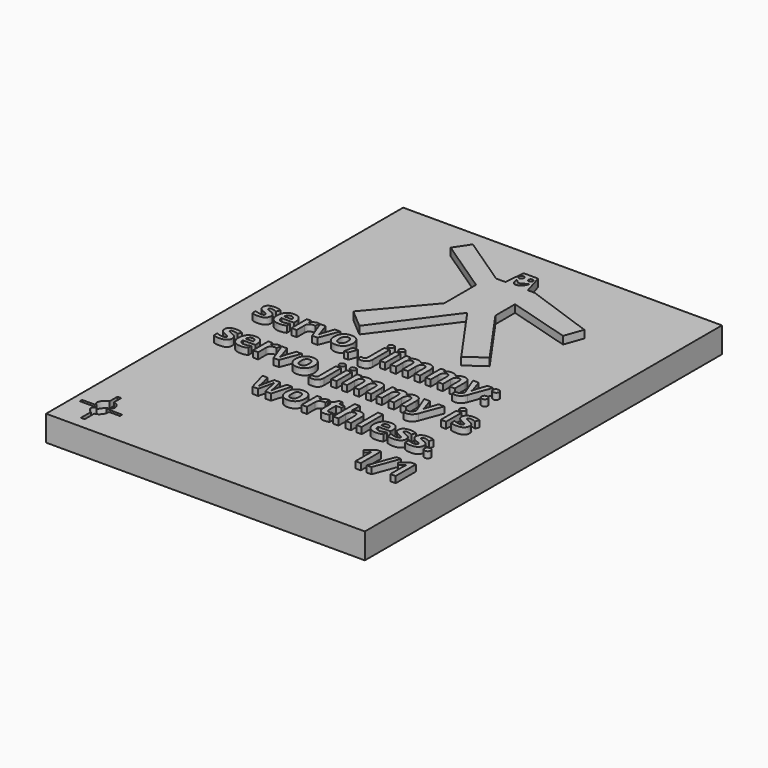
from build123d import *

# Parameters (mm, degrees)
F0_W         = 63.5
F0_H         = 88.9
F1_DEPTH     = 5.08
F2_R         = 0.483936804
F2_R_2       = 0.4231425129
F3_DEPTH     = 1.524
F5_DEPTH     = 1.27
F6_TEXT_SIZE = 7.0555555556
F7_DEPTH     = 1.27


# Not quite as in the source:
# - Text() gives the source's letters only with a copy of the font that has no kerning and outlines rounded to 1/6400 em; it was checked with that copy


with BuildPart() as f1:
    # F0 (on Top) → F1 (new body)
    with BuildSketch(Plane.XY):
        Rectangle(F0_W, F0_H)
    extrude(amount=F1_DEPTH)

    # F2 (on face) → F3 (join)
    with BuildSketch(Plane.XY.offset(5.08)):
        Polygon((-10.3656723576, 6.8217876206), (0, 20.7275711), (8.5247382522, 8.577182889), (12.1481206254, 11.1193556807), (4.0015474354, 22.7307417338), (4.0015474354, 27.6327357116), (4.0015474354, 32.5347296894), (2.6223212481, 32.5347296894), (0, 32.5347296894), (-1.8471479416, 32.5347296894), (-3.6942958832, 32.5347296894), (-13.7166529894, 39.2620638013), (-15.7326752015, 36.2586014777), (-4.7968987376, 28.9181503975), (-4.7968987376, 21.0021585226), (-14.1285285354, 10.0187547505), align=None)
        Polygon((4.0015474354, 32.5347296894), (4.0015474354, 27.6327357116), (16.4861305487, 23.9590620018), (17.7919864655, 27.6327357116), align=None)
        Polygon((0, 32.5347296894), (2.6223212481, 32.5347296894), (1.399056986, 36.6094112396), (0, 36.6094112396), (-1.4804843813, 36.6094112396), (-1.8471479416, 32.5347296894), align=None)
        with Locations((-0.8866756689, 35.3195294738)):
            Circle(F2_R, mode=Mode.SUBTRACT)
        with BuildLine():
            add(Edge.make_bspline(
                [(-0.8501152042, 34.1562442482), (-0.7343137138, 34.1961865805), (-0.0467516661, 32.880225173), (1.9143940204, 35.0437316808), (1.0316503155, 32.8797391223), (-0.7778123329, 32.509153736), (-0.9740249003, 34.1135052277), (-0.8501152042, 34.1562442482)],
                knots=[0, 0, 0, 0, 0.1780613573, 0.4016291559, 0.5959136983, 0.8094711166, 1, 1, 1, 1], degree=3))
        make_face(mode=Mode.SUBTRACT)
        with Locations((0.9081121534, 35.3893265128)):
            Circle(F2_R_2, mode=Mode.SUBTRACT)
    extrude(amount=F3_DEPTH)

    # F4 (on face) → F5 (cut)
    with BuildSketch(Plane.XY.offset(5.08)):
        with BuildLine():
            add(Edge.make_bspline(
                [(-25.6292883469, -37.4438245498), (-25.5440439647, -37.4063721569), (-25.4620471143, -37.3631067403), (-25.3843005295, -37.3148079962)],
                knots=[0.0680076943, 0.0680076943, 0.0680076943, 0.0680076943, 0.0966302435, 0.0966302435, 0.0966302435, 0.0966302435], degree=3))
            add(Edge.make_bspline(
                [(-25.6292883469, -37.4438245498), (-25.2227961776, -37.3837119487), (-24.7132209679, -37.4270308297), (-24.5209995881, -37.774670522), (-24.4905924923, -37.8889460117)],
                knots=[0.0689407267, 0.0689407267, 0.0689407267, 0.0689407267, 0.2018413649, 0.2544963619, 0.2544963619, 0.2544963619, 0.2544963619], degree=3))
            Line((-24.4905924923, -37.8889460117), (-22.2920402884, -37.8889460117))
            Line((-22.2920402884, -37.8889460117), (-22.2920402884, -37.3148079962))
            Line((-22.2920402884, -37.3148079962), (-25.3843005295, -37.3148079962))
        make_face()
        with BuildLine():
            Line((-26.6530141234, -37.5985746456), (-26.6530141234, -37.5851999525))
            add(Edge.make_bspline(
                [(-27.4060703076, -37.3148079962), (-27.1886195833, -37.4508936414), (-26.9254983415, -37.5462389939), (-26.6530141234, -37.5851999525)],
                knots=[0.8801095423, 0.8801095423, 0.8801095423, 0.8801095423, 0.9624938443, 0.9624938443, 0.9624938443, 0.9624938443], degree=3))
            Line((-27.4060703076, -37.3148079962), (-30.2648916841, -37.3148079962))
            Line((-30.2648916841, -37.3148079962), (-30.2648916841, -37.8889460117))
            Line((-30.2648916841, -37.8889460117), (-27.800713044, -37.8889460117))
            Line((-27.800713044, -37.8889460117), (-26.6530141234, -37.5985746456))
        make_face()
        with BuildLine():
            add(Edge.make_bspline(
                [(-25.867716277, -37.5305749744), (-25.7860798434, -37.5067937197), (-25.706356866, -37.4776848511), (-25.6292883469, -37.4438245498)],
                knots=[0.0421303588, 0.0421303588, 0.0421303588, 0.0421303588, 0.0680076943, 0.0680076943, 0.0680076943, 0.0680076943], degree=3))
            Line((-25.867716277, -37.5305749744), (-25.799085371, -37.8889460117))
            Line((-25.799085371, -37.8889460117), (-24.4905924923, -37.8889460117))
            add(Edge.make_bspline(
                [(-25.6292883469, -37.4438245498), (-25.2227961776, -37.3837119487), (-24.7132209679, -37.4270308297), (-24.5209995881, -37.774670522), (-24.4905924923, -37.8889460117)],
                knots=[0.0689407267, 0.0689407267, 0.0689407267, 0.0689407267, 0.2018413649, 0.2544963619, 0.2544963619, 0.2544963619, 0.2544963619], degree=3))
        make_face()
        with BuildLine():
            add(Edge.make_bspline(
                [(-26.2784659863, -37.6018770039), (-26.1512643353, -37.5946117228), (-26.0256129936, -37.5736079501), (-25.9039178491, -37.540736433)],
                knots=[0, 0, 0, 0, 0.0383181812, 0.0383181812, 0.0383181812, 0.0383181812], degree=3))
            add(Edge.make_bspline(
                [(-26.6530141234, -37.7449608069), (-26.5332231792, -37.6918141298), (-26.4068589747, -37.6441222626), (-26.2784659863, -37.6018770039)],
                knots=[0.9590736268, 0.9590736268, 0.9590736268, 0.9590736268, 1, 1, 1, 1], degree=3))
            Line((-26.6530141234, -37.7449608069), (-26.6530141234, -37.8889460117))
            Line((-26.6530141234, -37.8889460117), (-25.9039178491, -37.8889460117))
            Line((-25.9039178491, -37.8889460117), (-25.9039178491, -37.540736433))
        make_face()
        with BuildLine():
            add(Edge.make_bspline(
                [(-25.9039178491, -37.540736433), (-25.8918107112, -37.5374661301), (-25.8797427308, -37.5340783632), (-25.867716277, -37.5305749744)],
                knots=[0.0383181812, 0.0383181812, 0.0383181812, 0.0383181812, 0.0421303588, 0.0421303588, 0.0421303588, 0.0421303588], degree=3))
            Line((-25.9039178491, -37.540736433), (-25.9039178491, -37.8889460117))
            Line((-25.9039178491, -37.8889460117), (-25.799085371, -37.8889460117))
            Line((-25.799085371, -37.8889460117), (-25.867716277, -37.5305749744))
        make_face()
        with BuildLine():
            Line((-26.6530141234, -37.8889460117), (-26.6530141234, -37.7449608069))
            add(Edge.make_bspline(
                [(-26.9357420062, -37.8889460117), (-26.8477942788, -37.837171916), (-26.7526792421, -37.7891784222), (-26.6530141234, -37.7449608069)],
                knots=[0.9250232078, 0.9250232078, 0.9250232078, 0.9250232078, 0.9590736268, 0.9590736268, 0.9590736268, 0.9590736268], degree=3))
            Line((-26.9357420062, -37.8889460117), (-26.6530141234, -37.8889460117))
        make_face()
        with BuildLine():
            add(Edge.make_bspline(
                [(-26.9357420062, -37.8889460117), (-26.8477942788, -37.837171916), (-26.7526792421, -37.7891784222), (-26.6530141234, -37.7449608069)],
                knots=[0.9250232078, 0.9250232078, 0.9250232078, 0.9250232078, 0.9590736268, 0.9590736268, 0.9590736268, 0.9590736268], degree=3))
            Line((-26.6530141234, -37.7449608069), (-26.6530141234, -37.5985746456))
            Line((-26.6530141234, -37.5985746456), (-27.800713044, -37.8889460117))
            Line((-27.800713044, -37.8889460117), (-26.9357420062, -37.8889460117))
        make_face()
        with BuildLine():
            add(Edge.make_bspline(
                [(-26.6530141234, -37.7449608069), (-26.5332231792, -37.6918141298), (-26.4068589747, -37.6441222626), (-26.2784659863, -37.6018770039)],
                knots=[0.9590736268, 0.9590736268, 0.9590736268, 0.9590736268, 1, 1, 1, 1], degree=3))
            add(Edge.make_bspline(
                [(-26.6184572109, -37.5898316401), (-26.5056098451, -37.6039463068), (-26.391426612, -37.6083288911), (-26.2784659863, -37.6018770039)],
                knots=[0.9659717803, 0.9659717803, 0.9659717803, 0.9659717803, 1, 1, 1, 1], degree=3))
            Line((-26.6184572109, -37.5898316401), (-26.6530141234, -37.5985746456))
            Line((-26.6530141234, -37.5985746456), (-26.6530141234, -37.7449608069))
        make_face()
        with BuildLine():
            add(Edge.make_bspline(
                [(-26.6184572109, -37.5898316401), (-26.5056098451, -37.6039463068), (-26.391426612, -37.6083288911), (-26.2784659863, -37.6018770039)],
                knots=[0.9659717803, 0.9659717803, 0.9659717803, 0.9659717803, 1, 1, 1, 1], degree=3))
            add(Edge.make_bspline(
                [(-26.2784659863, -37.6018770039), (-26.1544455385, -37.5610704462), (-26.028532138, -37.5253458354), (-25.9039178491, -37.4964132695)],
                knots=[0, 0, 0, 0, 0.0395325881, 0.0395325881, 0.0395325881, 0.0395325881], degree=3))
            Line((-25.9039178491, -37.4964132695), (-25.9039178491, -37.4090509781))
            Line((-25.9039178491, -37.4090509781), (-26.6184572109, -37.5898316401))
        make_face()
        with BuildLine():
            add(Edge.make_bspline(
                [(-26.2784659863, -37.6018770039), (-26.1544455385, -37.5610704462), (-26.028532138, -37.5253458354), (-25.9039178491, -37.4964132695)],
                knots=[0, 0, 0, 0, 0.0395325881, 0.0395325881, 0.0395325881, 0.0395325881], degree=3))
            add(Edge.make_bspline(
                [(-26.2784659863, -37.6018770039), (-26.1512643353, -37.5946117228), (-26.0256129936, -37.5736079501), (-25.9039178491, -37.540736433)],
                knots=[0, 0, 0, 0, 0.0383181812, 0.0383181812, 0.0383181812, 0.0383181812], degree=3))
            Line((-25.9039178491, -37.540736433), (-25.9039178491, -37.4964132695))
        make_face()
        with BuildLine():
            Line((-25.8915865661, -37.4059311255), (-25.875500397, -37.4899285173))
            add(Edge.make_bspline(
                [(-25.875500397, -37.4899285173), (-25.7924251289, -37.4713036122), (-25.7100375443, -37.4557658482), (-25.6292883469, -37.4438245498)],
                knots=[0.0425401693, 0.0425401693, 0.0425401693, 0.0425401693, 0.0689407267, 0.0689407267, 0.0689407267, 0.0689407267], degree=3))
            add(Edge.make_bspline(
                [(-25.6292883469, -37.4438245498), (-25.5440439647, -37.4063721569), (-25.4620471143, -37.3631067403), (-25.3843005295, -37.3148079962)],
                knots=[0.0680076943, 0.0680076943, 0.0680076943, 0.0680076943, 0.0966302435, 0.0966302435, 0.0966302435, 0.0966302435], degree=3))
            Line((-25.3843005295, -37.3148079962), (-25.5314204842, -37.3148079962))
            Line((-25.5314204842, -37.3148079962), (-25.8915865661, -37.4059311255))
        make_face()
        with BuildLine():
            Line((-25.9039178491, -37.4090509781), (-25.9039178491, -37.4964132695))
            add(Edge.make_bspline(
                [(-25.9039178491, -37.4964132695), (-25.8944373773, -37.4942121225), (-25.8849644248, -37.4920502874), (-25.875500397, -37.4899285173)],
                knots=[0.0395325881, 0.0395325881, 0.0395325881, 0.0395325881, 0.0425401693, 0.0425401693, 0.0425401693, 0.0425401693], degree=3))
            Line((-25.875500397, -37.4899285173), (-25.8915865661, -37.4059311255))
            Line((-25.8915865661, -37.4059311255), (-25.9039178491, -37.4090509781))
        make_face()
        with BuildLine():
            Line((-25.875500397, -37.4899285173), (-25.867716277, -37.5305749744))
            add(Edge.make_bspline(
                [(-25.867716277, -37.5305749744), (-25.7860798434, -37.5067937197), (-25.706356866, -37.4776848511), (-25.6292883469, -37.4438245498)],
                knots=[0.0421303588, 0.0421303588, 0.0421303588, 0.0421303588, 0.0680076943, 0.0680076943, 0.0680076943, 0.0680076943], degree=3))
            add(Edge.make_bspline(
                [(-25.875500397, -37.4899285173), (-25.7924251289, -37.4713036122), (-25.7100375443, -37.4557658482), (-25.6292883469, -37.4438245498)],
                knots=[0.0425401693, 0.0425401693, 0.0425401693, 0.0425401693, 0.0689407267, 0.0689407267, 0.0689407267, 0.0689407267], degree=3))
        make_face()
        with BuildLine():
            Line((-25.9039178491, -37.4964132695), (-25.9039178491, -37.540736433))
            add(Edge.make_bspline(
                [(-25.9039178491, -37.540736433), (-25.8918107112, -37.5374661301), (-25.8797427308, -37.5340783632), (-25.867716277, -37.5305749744)],
                knots=[0.0383181812, 0.0383181812, 0.0383181812, 0.0383181812, 0.0421303588, 0.0421303588, 0.0421303588, 0.0421303588], degree=3))
            Line((-25.867716277, -37.5305749744), (-25.875500397, -37.4899285173))
            add(Edge.make_bspline(
                [(-25.9039178491, -37.4964132695), (-25.8944373773, -37.4942121225), (-25.8849644248, -37.4920502874), (-25.875500397, -37.4899285173)],
                knots=[0.0395325881, 0.0395325881, 0.0395325881, 0.0395325881, 0.0425401693, 0.0425401693, 0.0425401693, 0.0425401693], degree=3))
        make_face()
        with BuildLine():
            add(Edge.make_bspline(
                [(-27.4060703076, -37.3148079962), (-27.1886195833, -37.4508936414), (-26.9254983415, -37.5462389939), (-26.6530141234, -37.5851999525)],
                knots=[0.8801095423, 0.8801095423, 0.8801095423, 0.8801095423, 0.9624938443, 0.9624938443, 0.9624938443, 0.9624938443], degree=3))
            Line((-26.6530141234, -37.5851999525), (-26.6530141234, -37.3148079962))
            Line((-26.6530141234, -37.3148079962), (-27.4060703076, -37.3148079962))
        make_face()
        with BuildLine():
            Line((-26.6530141234, -37.5985746456), (-26.6184572109, -37.5898316401))
            add(Edge.make_bspline(
                [(-26.6530141234, -37.5851999525), (-26.6415109286, -37.5868447285), (-26.6299910472, -37.5883890167), (-26.6184572109, -37.5898316401)],
                knots=[0.9624938443, 0.9624938443, 0.9624938443, 0.9624938443, 0.9659717803, 0.9659717803, 0.9659717803, 0.9659717803], degree=3))
            Line((-26.6530141234, -37.5851999525), (-26.6530141234, -37.5985746456))
        make_face()
        Polygon((-25.9039178491, -37.3415406793), (-25.8915865661, -37.4059311255), (-25.5314204842, -37.3148079962), (-25.9039178491, -37.3148079962), align=None)
        Polygon((-25.9039178491, -37.3415406793), (-25.9039178491, -37.4090509781), (-25.8915865661, -37.4059311255), align=None)
        with BuildLine():
            add(Edge.make_bspline(
                [(-26.6530141234, -37.5851999525), (-26.6415109286, -37.5868447285), (-26.6299910472, -37.5883890167), (-26.6184572109, -37.5898316401)],
                knots=[0.9624938443, 0.9624938443, 0.9624938443, 0.9624938443, 0.9659717803, 0.9659717803, 0.9659717803, 0.9659717803], degree=3))
            Line((-26.6184572109, -37.5898316401), (-25.9039178491, -37.4090509781))
            Line((-25.9039178491, -37.4090509781), (-25.9039178491, -37.3415406793))
            Line((-25.9039178491, -37.3415406793), (-25.9090373707, -37.3148079962))
            Line((-25.9090373707, -37.3148079962), (-26.6530141234, -37.3148079962))
            Line((-26.6530141234, -37.3148079962), (-26.6530141234, -37.5851999525))
        make_face()
        Polygon((-25.9090373707, -37.3148079962), (-25.9039178491, -37.3415406793), (-25.9039178491, -37.3148079962), align=None)
        with BuildLine():
            Line((-26.6530141234, -33.4299733636), (-26.3738592999, -34.8876403164))
            add(Edge.make_bspline(
                [(-25.9039178491, -34.8487733214), (-25.9381402301, -34.8454654833), (-26.0912524955, -34.8370087275), (-26.250328173, -34.8573958338), (-26.3738592999, -34.8876403164)],
                knots=[0.4751565099, 0.4751565099, 0.4751565099, 0.4751565099, 0.4859384918, 0.5229046656, 0.5229046656, 0.5229046656, 0.5229046656], degree=3))
            Line((-25.9039178491, -34.8487733214), (-25.9039178491, -33.03899616))
            Line((-25.9039178491, -33.03899616), (-26.6530141234, -33.03899616))
            Line((-26.6530141234, -33.03899616), (-26.6530141234, -33.4299733636))
        make_face()
        with BuildLine():
            Line((-26.6530141234, -33.4299733636), (-26.6530141234, -34.9796937447))
            add(Edge.make_bspline(
                [(-26.3738592999, -34.8876403164), (-26.4671555366, -34.9104823034), (-26.5606663734, -34.9415727539), (-26.6530141234, -34.9796937447)],
                knots=[0.5229046656, 0.5229046656, 0.5229046656, 0.5229046656, 0.5508231747, 0.5508231747, 0.5508231747, 0.5508231747], degree=3))
            Line((-26.3738592999, -34.8876403164), (-26.6530141234, -33.4299733636))
        make_face()
        with BuildLine():
            Line((-26.3738592999, -34.8876403164), (-25.9090373707, -37.3148079962))
            Line((-25.9090373707, -37.3148079962), (-25.9039178491, -37.3148079962))
            Line((-25.9039178491, -37.3148079962), (-25.9039178491, -34.8487733214))
            add(Edge.make_bspline(
                [(-25.9039178491, -34.8487733214), (-25.9381402301, -34.8454654833), (-26.0912524955, -34.8370087275), (-26.250328173, -34.8573958338), (-26.3738592999, -34.8876403164)],
                knots=[0.4751565099, 0.4751565099, 0.4751565099, 0.4751565099, 0.4859384918, 0.5229046656, 0.5229046656, 0.5229046656, 0.5229046656], degree=3))
        make_face()
        with BuildLine():
            Line((-26.6530141234, -34.9796937447), (-26.6530141234, -37.3148079962))
            Line((-26.6530141234, -37.3148079962), (-25.9090373707, -37.3148079962))
            Line((-25.9090373707, -37.3148079962), (-26.3738592999, -34.8876403164))
            add(Edge.make_bspline(
                [(-26.3738592999, -34.8876403164), (-26.4671555366, -34.9104823034), (-26.5606663734, -34.9415727539), (-26.6530141234, -34.9796937447)],
                knots=[0.5229046656, 0.5229046656, 0.5229046656, 0.5229046656, 0.5508231747, 0.5508231747, 0.5508231747, 0.5508231747], degree=3))
        make_face()
        with BuildLine():
            Line((-25.9039178491, -39.7897740875), (-25.9039178491, -37.8889460117))
            Line((-25.9039178491, -37.8889460117), (-26.6530141234, -37.8889460117))
            Line((-26.6530141234, -37.8889460117), (-26.6530141234, -39.6745179496))
            add(Edge.make_bspline(
                [(-25.9039178491, -39.7897740875), (-26.0275826985, -39.8106109895), (-26.2811416622, -39.8159788988), (-26.5322915736, -39.7329578405), (-26.6530141234, -39.6745179496)],
                knots=[0.5533362898, 0.5533362898, 0.5533362898, 0.5533362898, 0.5952987557, 0.6379564705, 0.6379564705, 0.6379564705, 0.6379564705], degree=3))
        make_face()
        with BuildLine():
            Line((-25.9039178491, -42.1647578478), (-25.9039178491, -39.7897740875))
            add(Edge.make_bspline(
                [(-25.9039178491, -39.7897740875), (-26.0275826985, -39.8106109895), (-26.2811416622, -39.8159788988), (-26.5322915736, -39.7329578405), (-26.6530141234, -39.6745179496)],
                knots=[0.5533362898, 0.5533362898, 0.5533362898, 0.5533362898, 0.5952987557, 0.6379564705, 0.6379564705, 0.6379564705, 0.6379564705], degree=3))
            Line((-26.6530141234, -39.6745179496), (-26.6530141234, -42.1647578478))
            Line((-26.6530141234, -42.1647578478), (-25.9039178491, -42.1647578478))
        make_face()
        with BuildLine():
            Line((-26.6530141234, -37.8889460117), (-26.9357420062, -37.8889460117))
            add(Edge.make_bspline(
                [(-26.6530141234, -39.6745179496), (-27.1164712396, -39.4501656364), (-27.7768621542, -38.6283352298), (-27.2542163688, -38.0764292201), (-26.9357420062, -37.8889460117)],
                knots=[0.6379564705, 0.6379564705, 0.6379564705, 0.6379564705, 0.8017205847, 0.9250232078, 0.9250232078, 0.9250232078, 0.9250232078], degree=3))
            Line((-26.6530141234, -39.6745179496), (-26.6530141234, -37.8889460117))
        make_face()
        with BuildLine():
            Line((-25.799085371, -37.8889460117), (-25.9039178491, -37.8889460117))
            Line((-25.9039178491, -37.8889460117), (-25.9039178491, -39.7897740875))
            add(Edge.make_bspline(
                [(-25.4641004909, -39.6381416131), (-25.6043449244, -39.7115548228), (-25.7525790829, -39.7642742704), (-25.9039178491, -39.7897740875)],
                knots=[0.5019833965, 0.5019833965, 0.5019833965, 0.5019833965, 0.5533362898, 0.5533362898, 0.5533362898, 0.5533362898], degree=3))
            Line((-25.4641004909, -39.6381416131), (-25.799085371, -37.8889460117))
        make_face()
        with BuildLine():
            Line((-24.4905924923, -37.8889460117), (-25.799085371, -37.8889460117))
            Line((-25.799085371, -37.8889460117), (-25.4641004909, -39.6381416131))
            add(Edge.make_bspline(
                [(-24.4905924923, -37.8889460117), (-24.4194242045, -38.1564095991), (-24.5420591138, -38.8654216274), (-25.1247822027, -39.4605199849), (-25.4641004909, -39.6381416131)],
                knots=[0.2544963619, 0.2544963619, 0.2544963619, 0.2544963619, 0.3777362133, 0.5019833965, 0.5019833965, 0.5019833965, 0.5019833965], degree=3))
        make_face()
        with BuildLine():
            add(Edge.make_bspline(
                [(-26.6530141234, -34.9796937447), (-27.33957535, -35.2631050268), (-28.3267884635, -36.3292110728), (-27.7273612416, -37.1137367686), (-27.4060703076, -37.3148079962)],
                knots=[0.5508231747, 0.5508231747, 0.5508231747, 0.5508231747, 0.7583838989, 0.8801095423, 0.8801095423, 0.8801095423, 0.8801095423], degree=3))
            Line((-27.4060703076, -37.3148079962), (-26.6530141234, -37.3148079962))
            Line((-26.6530141234, -37.3148079962), (-26.6530141234, -34.9796937447))
        make_face()
        with BuildLine():
            Line((-25.9039178491, -37.3148079962), (-25.5314204842, -37.3148079962))
            Line((-25.5314204842, -37.3148079962), (-25.2931777962, -37.2545318614))
            add(Edge.make_bspline(
                [(-25.2931777962, -37.2545318614), (-24.9299751093, -36.9989898731), (-24.2705243879, -36.0330893249), (-25.1835388986, -34.9184031027), (-25.9039178491, -34.8487733214)],
                knots=[0.1080704067, 0.1080704067, 0.1080704067, 0.1080704067, 0.2481964756, 0.4751565099, 0.4751565099, 0.4751565099, 0.4751565099], degree=3))
            Line((-25.9039178491, -34.8487733214), (-25.9039178491, -37.3148079962))
        make_face()
        with BuildLine():
            Line((-25.5314204842, -37.3148079962), (-25.3843005295, -37.3148079962))
            add(Edge.make_bspline(
                [(-25.3843005295, -37.3148079962), (-25.3532259523, -37.2955034433), (-25.3228303658, -37.2753948034), (-25.2931777962, -37.2545318614)],
                knots=[0.0966302435, 0.0966302435, 0.0966302435, 0.0966302435, 0.1080704067, 0.1080704067, 0.1080704067, 0.1080704067], degree=3))
            Line((-25.2931777962, -37.2545318614), (-25.5314204842, -37.3148079962))
        make_face()
    extrude(amount=-F5_DEPTH, mode=Mode.SUBTRACT)

    # F6 (on face) → F7 (join)
    with BuildSketch(Plane.XY.offset(5.08)):
        with Locations((-26.67, 0)):
            Text('servo, jimmy:', F6_TEXT_SIZE, font='Open Sans', font_style=FontStyle.BOLD, text_align=(TextAlign.LEFT, TextAlign.BOTTOM))
        with Locations((-26.67, -9.5955555556)):
            Text('servo jimmy is', F6_TEXT_SIZE, font='Open Sans', font_style=FontStyle.BOLD, text_align=(TextAlign.LEFT, TextAlign.BOTTOM))
        with Locations((-12.0032638889, -19.1911111111)):
            Text('worthless.', F6_TEXT_SIZE, font='Open Sans', font_style=FontStyle.BOLD, text_align=(TextAlign.LEFT, TextAlign.BOTTOM))
        with Locations((15.4968663194, -28.7866666667)):
            Text('1/1', F6_TEXT_SIZE, font='Open Sans', font_style=FontStyle.BOLD, text_align=(TextAlign.LEFT, TextAlign.BOTTOM))
    extrude(amount=F7_DEPTH)


solid = f1.part
